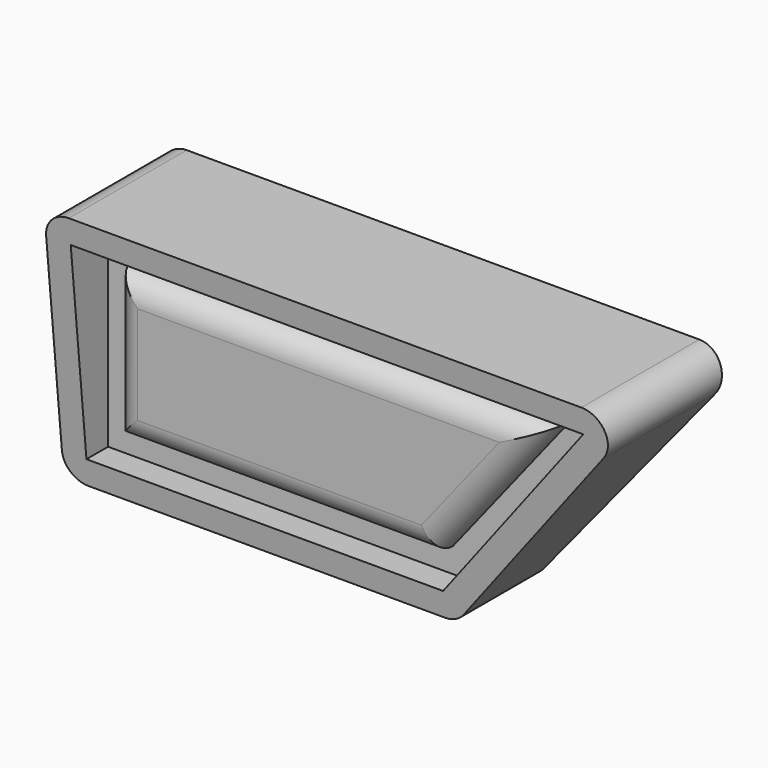
from build123d import *

# Parameters (mm, degrees)
F2_DEPTH      = 120
F4_DEPTH      = 15.001
F4_DEPTH_BACK = 15.001
F6_DEPTH      = 25
F8_DEPTH      = 5
F9_R          = 4.99999
F11_R         = 5


# Not quite as in the source:
# - a fillet or chamfer is up to 0.001 mm smaller than in the source, because OpenCascade refuses the exact size
# - a pattern or mirror of a feature is missing from the dataset's text; its kind, count and spacing are read off the source's solid


with BuildPart() as f2:
    # F1 (on Right) → F2 (new body)
    with BuildSketch(Plane.YZ):
        Polygon((-10, 0), (0, 0), (10, 0), (15, 50), (0, 50), (-15, 50), align=None)
    extrude(amount=F2_DEPTH)

    # F3 (on Front) → F4 (cut, two sides)
    with BuildSketch(Plane.XZ) as f4_sk:
        Polygon((120, 50.4512232197), (80, 0), (120, 0), align=None)
    extrude(amount=-F4_DEPTH, mode=Mode.SUBTRACT)
    extrude(f4_sk.sketch, amount=F4_DEPTH_BACK, mode=Mode.SUBTRACT)

    # F5 (on offset) → F6 (cut)
    with BuildSketch(Plane.XZ.offset(5)):
        Polygon((5, 45), (5, 5), (77.5833880732, 5), (109.2971880149, 45), align=None)
    f6 = extrude(amount=F6_DEPTH, mode=Mode.SUBTRACT)

    # F6_copies: F6 across plane
    add(f6.mirror(Plane.ZX), mode=Mode.SUBTRACT)

    # F11
    f11_edges = [f2.edges().sort_by_distance(p)[0] for p in [
        (119.64225, 0, 50),
        (80, 0, 0),
        (0, 0, 0),
        (0, 0, 50),
    ]]
    fillet(f11_edges, radius=F11_R)


with BuildPart() as f8:
    # F7 (on face) → F8 (new body)
    with BuildSketch(Plane.XZ.offset(5)):
        Polygon((10, 40), (10, 10), (75.1667761465, 10), (98.9521261027, 40), align=None)
    extrude(amount=F8_DEPTH)

    # F9 (radius 5 in the source; OpenCascade refuses exactly that, so slightly less here)
    f9_edges = [f8.edges().sort_by_distance(p)[0] for p in [
        (10, -10, 25),
        (42.583388, -10, 10),
        (87.059451, -10, 25),
        (54.476063, -10, 40),
    ]]
    fillet(f9_edges, radius=F9_R)


with BuildPart() as f10_1:
    # F10: instance of F8
    add(f8.part.mirror(Plane.XZ))


solid = Compound([f2.part, f8.part, f10_1.part])
